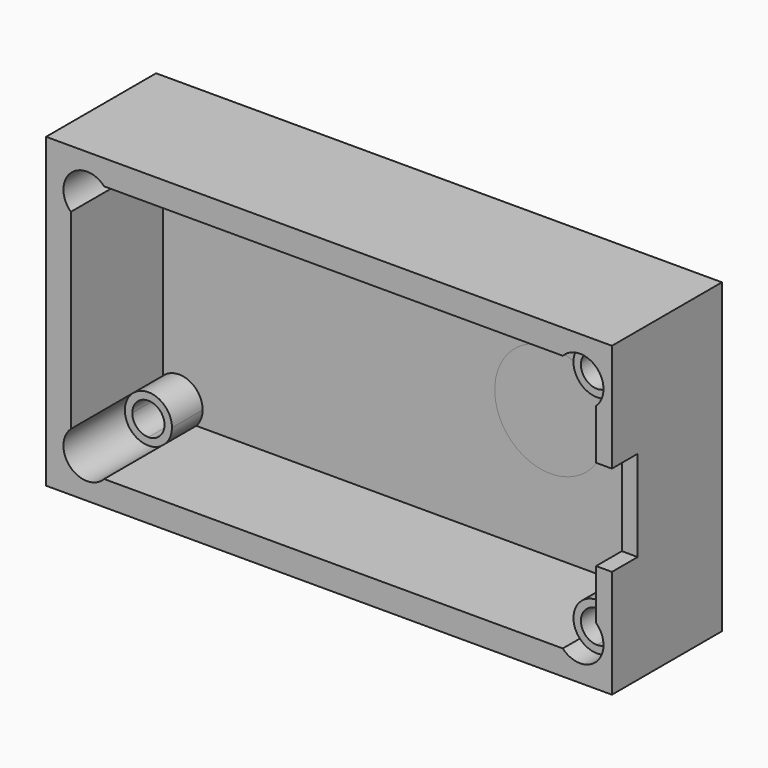
from build123d import *

# Parameters (mm, degrees)
F0_W     = 22.84
F0_H     = 12.4
F1_DEPTH = 5.55
F0_R     = 2.25
F2_DEPTH = 0.9
F3_DEPTH = 4.69
F4_DEPTH = 2.45
F5_W     = 1.3
F5_H     = 3.67
F6_DEPTH = 1
F7_DEPTH = 0.9
F8_DEPTH = 3.06


# Not quite as in the source:
# - a feature names something its author has since deleted; it is built from what else it names


with BuildPart() as f1:
    # F0 (on Front) → F1 (new body)
    with BuildSketch(Plane.XZ):
        Rectangle(F0_W, F0_H)
        with BuildLine():
            ThreePointArc((11.08, 4.55), (11.0017797887, 4.1725082782), (10.78, 3.857179677))
            Line((10.78, 3.857179677), (10.78, -3.857179677))
            ThreePointArc((10.78, -3.857179677), (11.0017797887, -4.1725082782), (11.08, -4.55))
            ThreePointArc((11.08, -4.55), (10.479514444, -5.4333683566), (9.437179677, -5.2))
            Line((9.437179677, -5.2), (-9.077179677, -5.2))
            ThreePointArc((-9.077179677, -5.2), (-10.4417514421, -5.2217514421), (-10.42, -3.857179677))
            Line((-10.42, -3.857179677), (-10.42, 3.857179677))
            ThreePointArc((-10.42, 3.857179677), (-10.4417514421, 5.2217514421), (-9.077179677, 5.2))
            Line((-9.077179677, 5.2), (9.437179677, 5.2))
            ThreePointArc((9.437179677, 5.2), (10.479514444, 5.4333683566), (11.08, 4.55))
        make_face(mode=Mode.SUBTRACT)
    extrude(amount=F1_DEPTH)

    # F0 (on Front) → F2 (join)
    with BuildSketch(Plane.XZ):
        with BuildLine():
            Line((10.78, -3.857179677), (10.78, 3.857179677))
            ThreePointArc((10.78, 3.857179677), (9.4582485579, 3.8782485579), (9.437179677, 5.2))
            Line((9.437179677, 5.2), (-9.077179677, 5.2))
            ThreePointArc((-9.077179677, 5.2), (-8.8866316434, 4.899514444), (-8.82, 4.55))
            ThreePointArc((-8.82, 4.55), (-9.3925082782, 3.6782202113), (-10.42, 3.857179677))
            Line((-10.42, 3.857179677), (-10.42, -3.857179677))
            ThreePointArc((-10.42, -3.857179677), (-9.3925082782, -3.6782202113), (-8.82, -4.55))
            ThreePointArc((-8.82, -4.55), (-8.8866316434, -4.899514444), (-9.077179677, -5.2))
            Line((-9.077179677, -5.2), (9.437179677, -5.2))
            ThreePointArc((9.437179677, -5.2), (9.4582485579, -3.8782485579), (10.78, -3.857179677))
        make_face()
        with Locations((5.22, 0)):
            Circle(F0_R, mode=Mode.SUBTRACT)
    extrude(amount=F2_DEPTH)

    # F0 (on Front) → F3 (join)
    with BuildSketch(Plane.XZ):
        with BuildLine():
            Line((10.78, 3.857179677), (10.78, 4.55))
            ThreePointArc((10.78, 4.55), (9.6703805922, 4.0903805922), (10.13, 5.2))
            Line((10.13, 5.2), (9.437179677, 5.2))
            ThreePointArc((9.437179677, 5.2), (9.4582485579, 3.8782485579), (10.78, 3.857179677))
        make_face()
        with BuildLine():
            ThreePointArc((10.13, 5.2), (10.5896194078, 5.0096194078), (10.78, 4.55))
            Line((10.78, 4.55), (10.78, 3.857179677))
            ThreePointArc((10.78, 3.857179677), (11.0017797887, 4.1725082782), (11.08, 4.55))
            ThreePointArc((11.08, 4.55), (10.479514444, 5.4333683566), (9.437179677, 5.2))
            Line((9.437179677, 5.2), (10.13, 5.2))
        make_face()
        with BuildLine():
            Line((10.78, -4.55), (10.78, -3.857179677))
            ThreePointArc((10.78, -3.857179677), (9.4582485579, -3.8782485579), (9.437179677, -5.2))
            Line((9.437179677, -5.2), (10.13, -5.2))
            ThreePointArc((10.13, -5.2), (9.6703805922, -4.0903805922), (10.78, -4.55))
        make_face()
        with BuildLine():
            ThreePointArc((11.08, -4.55), (11.0017797887, -4.1725082782), (10.78, -3.857179677))
            Line((10.78, -3.857179677), (10.78, -4.55))
            ThreePointArc((10.78, -4.55), (10.5896194078, -5.0096194078), (10.13, -5.2))
            Line((10.13, -5.2), (9.437179677, -5.2))
            ThreePointArc((9.437179677, -5.2), (10.479514444, -5.4333683566), (11.08, -4.55))
        make_face()
    extrude(amount=F3_DEPTH)

    # F0 (on Front) → F4 (join)
    with BuildSketch(Plane.XZ):
        with BuildLine():
            Line((-9.77, 5.2), (-9.077179677, 5.2))
            ThreePointArc((-9.077179677, 5.2), (-10.4417514421, 5.2217514421), (-10.42, 3.857179677))
            Line((-10.42, 3.857179677), (-10.42, 4.55))
            ThreePointArc((-10.42, 4.55), (-10.2296194078, 5.0096194078), (-9.77, 5.2))
        make_face()
        with BuildLine():
            ThreePointArc((-8.82, 4.55), (-8.8866316434, 4.899514444), (-9.077179677, 5.2))
            Line((-9.077179677, 5.2), (-9.77, 5.2))
            ThreePointArc((-9.77, 5.2), (-9.3103805922, 5.0096194078), (-9.12, 4.55))
            ThreePointArc((-9.12, 4.55), (-9.77, 3.9), (-10.42, 4.55))
            Line((-10.42, 4.55), (-10.42, 3.857179677))
            ThreePointArc((-10.42, 3.857179677), (-9.3925082782, 3.6782202113), (-8.82, 4.55))
        make_face()
        with BuildLine():
            ThreePointArc((-10.42, -3.857179677), (-10.4417514421, -5.2217514421), (-9.077179677, -5.2))
            Line((-9.077179677, -5.2), (-9.77, -5.2))
            ThreePointArc((-9.77, -5.2), (-10.2296194078, -5.0096194078), (-10.42, -4.55))
            Line((-10.42, -4.55), (-10.42, -3.857179677))
        make_face()
        with BuildLine():
            Line((-9.77, -5.2), (-9.077179677, -5.2))
            ThreePointArc((-9.077179677, -5.2), (-8.8866316434, -4.899514444), (-8.82, -4.55))
            ThreePointArc((-8.82, -4.55), (-9.3925082782, -3.6782202113), (-10.42, -3.857179677))
            Line((-10.42, -3.857179677), (-10.42, -4.55))
            ThreePointArc((-10.42, -4.55), (-9.77, -3.9), (-9.12, -4.55))
            ThreePointArc((-9.12, -4.55), (-9.3103805922, -5.0096194078), (-9.77, -5.2))
        make_face()
    extrude(amount=F4_DEPTH)

    # F5 (on face) → F6 (cut)
    with BuildSketch(Plane.YZ.offset(11.42)):
        with Locations((-4.9, 0)):
            Rectangle(F5_W, F5_H)
    extrude(amount=-F6_DEPTH, mode=Mode.SUBTRACT)


with BuildPart() as f7:
    # F0 (on Front) → F7 (new body)
    with BuildSketch(Plane.XZ):
        with Locations((5.22, 0)):
            Circle(F0_R)
    extrude(amount=F7_DEPTH)

    # F8 (add): a face of the model
    f8_faces = [f7.faces().sort_by_distance(p)[0] for p in [
        (5.22, -0.9, 0),
    ]]
    extrude(f8_faces, amount=-F8_DEPTH)


solid = Compound([f1.part, f7.part])
